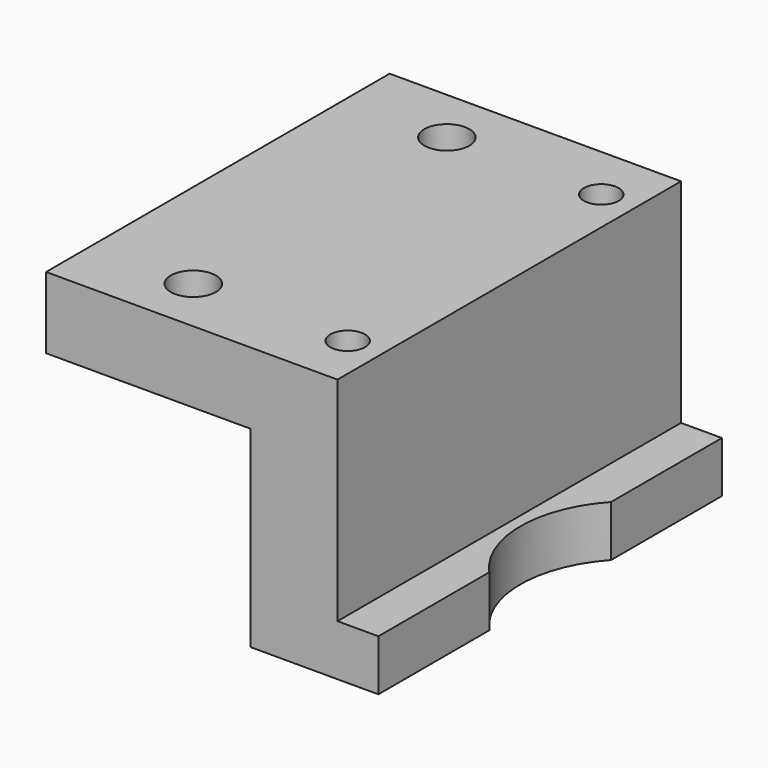
from build123d import *

# Parameters (mm, degrees)
F1_DEPTH     = 42
F2_R         = 1.7
F2_R_2       = 11
F3_DEPTH     = 25.801
F4_W         = 42
F4_H         = 7
F5_DEPTH     = 20
F6_R         = 2.2
F7_DEPTH     = 25
F8_TEXT_SIZE = 39.5833333333
F9_DEPTH     = 1
F10_DEPTH    = 1


# Not quite as in the source:
# - Text() gives the source's letters only with a copy of the font that has no kerning and outlines rounded to 1/6400 em; it was checked with that copy


with BuildPart() as f1:
    # F0 (on Front) → F1 (new body)
    with BuildSketch(Plane.XZ):
        Polygon((8.5, 5), (8.5, 25.8), (0, 25.8), (0, 0), (12.5, 0), (12.5, 5), align=None)
    extrude(amount=-F1_DEPTH)

    # F2 (on face) → F3 (cut, through all)
    with BuildSketch(Plane(origin=(0, 0, 0), x_dir=(1, 0, 0), z_dir=(0, 0, -1))):
        with Locations((5.1, -5.5)):
            Circle(F2_R)
        with Locations((5.1, -36.5)):
            Circle(F2_R)
        with Locations((20.6, -21)):
            Circle(F2_R_2)
    extrude(amount=-F3_DEPTH, mode=Mode.SUBTRACT)

    # F4 (on face) → F5 (join)
    with BuildSketch(Plane(origin=(0, 0, 0), x_dir=(0, -1, 0), z_dir=(-1, 0, 0))):
        with Locations((-21, 22.3)):
            Rectangle(F4_W, F4_H)
    extrude(amount=F5_DEPTH)

    # F6 (on face) → F7 (cut)
    with BuildSketch(Plane.XY.offset(25.8)):
        with Locations((-10, 36.5)):
            Circle(F6_R)
        with Locations((-10, 5.5)):
            Circle(F6_R)
    extrude(amount=-F7_DEPTH, mode=Mode.SUBTRACT)

    # F8 (on face) → F9 (join)
    with BuildSketch(Plane.XY.offset(25.8)):
        with Locations(Location((-20, 34.0655924479), (0, 0, -90))):
            Text('R', F8_TEXT_SIZE, font='Open Sans', font_style=FontStyle.BOLD, text_align=(TextAlign.LEFT, TextAlign.BOTTOM))
    extrude(amount=F9_DEPTH)

    # F10 (cut): a face of the model
    f10_faces = [f1.faces().sort_by_distance(p)[0] for p in [
        (-5.2937331808, 21.4303093571, 26.8),
    ]]
    extrude(f10_faces, amount=-F10_DEPTH, mode=Mode.SUBTRACT)


solid = f1.part
